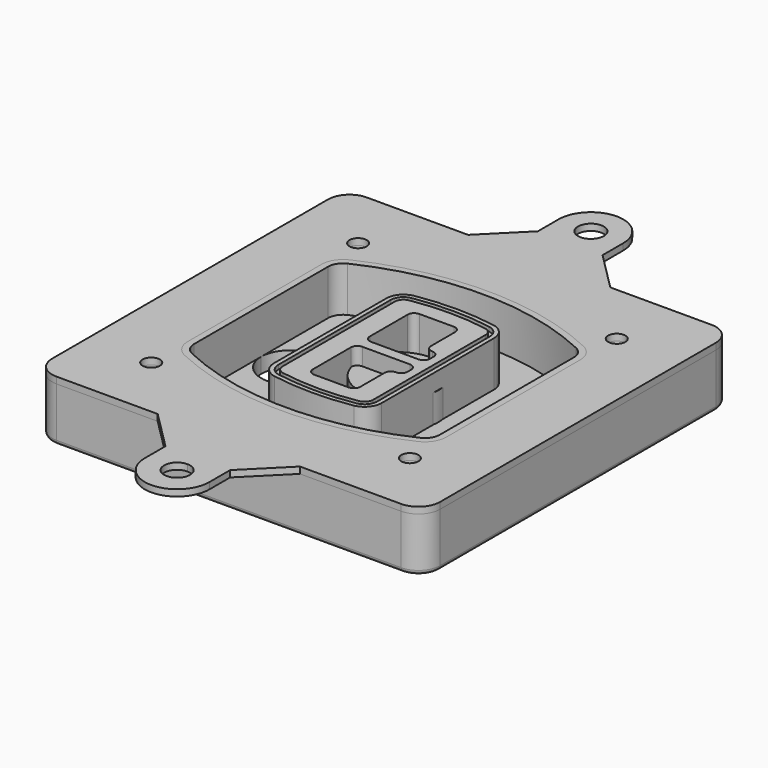
from build123d import *

# Parameters (mm, degrees)
F0_R      = 4
F1_DEPTH  = 25
F2_DEPTH  = 3
F3_DEPTH  = 18
F5_DEPTH  = 21
F6_DEPTH  = 2
F8_DEPTH  = 20
F9_DEPTH  = 16
F10_DEPTH = 25
F7_R      = 6
F7_R_2    = 4
F11_DEPTH = 6
F13_DEPTH = 9
F15_R     = 2
F16_R     = 6
F16_R_2   = 4
F17_DEPTH = 3


# Not quite as in the source:
# - a feature of the source that left no trace in its solid (it failed there, or was rolled back) is left out
# - a feature names something its author has since deleted; it is built from what else it names


with BuildPart() as f1:
    # F0 (on Top) → F1 (new body)
    with BuildSketch(Plane.XY):
        with BuildLine():
            ThreePointArc((-90, -80), (-87.0710678119, -87.0710678119), (-80, -90))
            Line((-80, -90), (80, -90))
            ThreePointArc((80, -90), (87.0710678119, -87.0710678119), (90, -80))
            Line((90, -80), (90, 80))
            ThreePointArc((90, 80), (87.0710678119, 87.0710678119), (80, 90))
            Line((80, 90), (-80, 90))
            ThreePointArc((-80, 90), (-87.0710678119, 87.0710678119), (-90, 80))
            Line((-90, 80), (-90, -80))
        make_face()
        with Locations((-60, -60)):
            Circle(F0_R, mode=Mode.SUBTRACT)
        with Locations((60, -60)):
            Circle(F0_R, mode=Mode.SUBTRACT)
        with Locations((-60, 60)):
            Circle(F0_R, mode=Mode.SUBTRACT)
        with BuildLine():
            ThreePointArc((-64, 38.8308515907), (-61.8195654598, 46.3340424013), (-55.9574468085, 51.5000594398))
            ThreePointArc((-55.9574468085, 51.5000594398), (0, 64), (55.9574468085, 51.5000594398))
            ThreePointArc((55.9574468085, 51.5000594398), (61.8195654598, 46.3340424013), (64, 38.8308515907))
            Line((64, 38.8308515907), (64, -38.8308515907))
            ThreePointArc((64, -38.8308515907), (61.8195654598, -46.3340424013), (55.9574468085, -51.5000594398))
            ThreePointArc((55.9574468085, -51.5000594398), (0, -64), (-55.9574468085, -51.5000594398))
            ThreePointArc((-55.9574468085, -51.5000594398), (-61.8195654598, -46.3340424013), (-64, -38.8308515907))
            Line((-64, -38.8308515907), (-64, 38.8308515907))
        make_face(mode=Mode.SUBTRACT)
        with Locations((60, 60)):
            Circle(F0_R, mode=Mode.SUBTRACT)
        with BuildLine():
            ThreePointArc((55.9574468085, 51.5000594398), (0, 64), (-55.9574468085, 51.5000594398))
            ThreePointArc((-55.9574468085, 51.5000594398), (-61.8195654598, 46.3340424013), (-64, 38.8308515907))
            Line((-64, 38.8308515907), (-64, -38.8308515907))
            ThreePointArc((-64, -38.8308515907), (-61.8195654598, -46.3340424013), (-55.9574468085, -51.5000594398))
            ThreePointArc((-55.9574468085, -51.5000594398), (0, -64), (55.9574468085, -51.5000594398))
            ThreePointArc((55.9574468085, -51.5000594398), (61.8195654598, -46.3340424013), (64, -38.8308515907))
            Line((64, -38.8308515907), (64, 38.8308515907))
            ThreePointArc((64, 38.8308515907), (61.8195654598, 46.3340424013), (55.9574468085, 51.5000594398))
        make_face()
        with BuildLine():
            Line((-60, -38.8308515907), (-60, 38.8308515907))
            ThreePointArc((-60, 38.8308515907), (-58.442546757, 44.1902735983), (-54.2553191489, 47.8802857686))
            ThreePointArc((-54.2553191489, 47.8802857686), (0, 60), (54.2553191489, 47.8802857686))
            ThreePointArc((54.2553191489, 47.8802857686), (58.442546757, 44.1902735983), (60, 38.8308515907))
            Line((60, 38.8308515907), (60, -38.8308515907))
            ThreePointArc((60, -38.8308515907), (58.442546757, -44.1902735983), (54.2553191489, -47.8802857686))
            ThreePointArc((54.2553191489, -47.8802857686), (0, -60), (-54.2553191489, -47.8802857686))
            ThreePointArc((-54.2553191489, -47.8802857686), (-58.442546757, -44.1902735983), (-60, -38.8308515907))
        make_face(mode=Mode.SUBTRACT)
        with BuildLine():
            ThreePointArc((-54.2553191489, 47.8802857686), (-58.442546757, 44.1902735983), (-60, 38.8308515907))
            Line((-60, 38.8308515907), (-60, -38.8308515907))
            ThreePointArc((-60, -38.8308515907), (-58.442546757, -44.1902735983), (-54.2553191489, -47.8802857686))
            ThreePointArc((-54.2553191489, -47.8802857686), (0, -60), (54.2553191489, -47.8802857686))
            ThreePointArc((54.2553191489, -47.8802857686), (58.442546757, -44.1902735983), (60, -38.8308515907))
            Line((60, -38.8308515907), (60, 38.8308515907))
            ThreePointArc((60, 38.8308515907), (58.442546757, 44.1902735983), (54.2553191489, 47.8802857686))
            ThreePointArc((54.2553191489, 47.8802857686), (0, 60), (-54.2553191489, 47.8802857686))
        make_face()
        with BuildLine():
            ThreePointArc((52.9787234043, 45.1654555152), (55.9097827299, 42.582446996), (57, 38.8308515907))
            Line((57, 38.8308515907), (57, -38.8308515907))
            ThreePointArc((57, -38.8308515907), (55.9097827299, -42.582446996), (52.9787234043, -45.1654555152))
            ThreePointArc((52.9787234043, -45.1654555152), (0, -57), (-52.9787234043, -45.1654555152))
            ThreePointArc((-52.9787234043, -45.1654555152), (-55.9097827299, -42.582446996), (-57, -38.8308515907))
            Line((-57, -38.8308515907), (-57, 38.8308515907))
            ThreePointArc((-57, 38.8308515907), (-55.9097827299, 42.582446996), (-52.9787234043, 45.1654555152))
            ThreePointArc((-52.9787234043, 45.1654555152), (0, 57), (52.9787234043, 45.1654555152))
        make_face(mode=Mode.SUBTRACT)
        with BuildLine():
            Line((57, -38.8308515907), (57, 38.8308515907))
            ThreePointArc((57, 38.8308515907), (55.9097827299, 42.582446996), (52.9787234043, 45.1654555152))
            ThreePointArc((52.9787234043, 45.1654555152), (0, 57), (-52.9787234043, 45.1654555152))
            ThreePointArc((-52.9787234043, 45.1654555152), (-55.9097827299, 42.582446996), (-57, 38.8308515907))
            Line((-57, 38.8308515907), (-57, -38.8308515907))
            ThreePointArc((-57, -38.8308515907), (-55.9097827299, -42.582446996), (-52.9787234043, -45.1654555152))
            ThreePointArc((-52.9787234043, -45.1654555152), (0, -57), (52.9787234043, -45.1654555152))
            ThreePointArc((52.9787234043, -45.1654555152), (55.9097827299, -42.582446996), (57, -38.8308515907))
        make_face()
    extrude(amount=-F1_DEPTH)

    # F0 (on Top) → F2 (join)
    with BuildSketch(Plane.XY):
        with BuildLine():
            ThreePointArc((-54.2553191489, 47.8802857686), (-58.442546757, 44.1902735983), (-60, 38.8308515907))
            Line((-60, 38.8308515907), (-60, -38.8308515907))
            ThreePointArc((-60, -38.8308515907), (-58.442546757, -44.1902735983), (-54.2553191489, -47.8802857686))
            ThreePointArc((-54.2553191489, -47.8802857686), (0, -60), (54.2553191489, -47.8802857686))
            ThreePointArc((54.2553191489, -47.8802857686), (58.442546757, -44.1902735983), (60, -38.8308515907))
            Line((60, -38.8308515907), (60, 38.8308515907))
            ThreePointArc((60, 38.8308515907), (58.442546757, 44.1902735983), (54.2553191489, 47.8802857686))
            ThreePointArc((54.2553191489, 47.8802857686), (0, 60), (-54.2553191489, 47.8802857686))
        make_face()
        with BuildLine():
            ThreePointArc((52.9787234043, 45.1654555152), (55.9097827299, 42.582446996), (57, 38.8308515907))
            Line((57, 38.8308515907), (57, -38.8308515907))
            ThreePointArc((57, -38.8308515907), (55.9097827299, -42.582446996), (52.9787234043, -45.1654555152))
            ThreePointArc((52.9787234043, -45.1654555152), (0, -57), (-52.9787234043, -45.1654555152))
            ThreePointArc((-52.9787234043, -45.1654555152), (-55.9097827299, -42.582446996), (-57, -38.8308515907))
            Line((-57, -38.8308515907), (-57, 38.8308515907))
            ThreePointArc((-57, 38.8308515907), (-55.9097827299, 42.582446996), (-52.9787234043, 45.1654555152))
            ThreePointArc((-52.9787234043, 45.1654555152), (0, 57), (52.9787234043, 45.1654555152))
        make_face(mode=Mode.SUBTRACT)
    extrude(amount=F2_DEPTH)

    # F0 (on Top) → F3 (cut)
    with BuildSketch(Plane.XY):
        with BuildLine():
            Line((57, -38.8308515907), (57, 38.8308515907))
            ThreePointArc((57, 38.8308515907), (55.9097827299, 42.582446996), (52.9787234043, 45.1654555152))
            ThreePointArc((52.9787234043, 45.1654555152), (0, 57), (-52.9787234043, 45.1654555152))
            ThreePointArc((-52.9787234043, 45.1654555152), (-55.9097827299, 42.582446996), (-57, 38.8308515907))
            Line((-57, 38.8308515907), (-57, -38.8308515907))
            ThreePointArc((-57, -38.8308515907), (-55.9097827299, -42.582446996), (-52.9787234043, -45.1654555152))
            ThreePointArc((-52.9787234043, -45.1654555152), (0, -57), (52.9787234043, -45.1654555152))
            ThreePointArc((52.9787234043, -45.1654555152), (55.9097827299, -42.582446996), (57, -38.8308515907))
        make_face()
    extrude(amount=-F3_DEPTH, mode=Mode.SUBTRACT)

    # F4 (on face) → F5 (join, through all)
    with BuildSketch(Plane.XY.offset(3)):
        with BuildLine():
            ThreePointArc((-25, -32.5662280692), (-23.1122504785, -37.7276614059), (-18.3399014778, -40.4532214146))
            ThreePointArc((-18.3399014778, -40.4532214146), (0, -42), (18.3399014778, -40.4532214146))
            ThreePointArc((18.3399014778, -40.4532214146), (23.1122504785, -37.7276614059), (25, -32.5662280692))
            Line((25, -32.5662280692), (25, 32.5662280692))
            ThreePointArc((25, 32.5662280692), (23.1122504785, 37.7276614059), (18.3399014778, 40.4532214146))
            ThreePointArc((18.3399014778, 40.4532214146), (0, 42), (-18.3399014778, 40.4532214146))
            ThreePointArc((-18.3399014778, 40.4532214146), (-23.1122504785, 37.7276614059), (-25, 32.5662280692))
            Line((-25, 32.5662280692), (-25, -32.5662280692))
        make_face()
        with BuildLine():
            ThreePointArc((18.0049261084, 38.4814730782), (21.5841878588, 36.4373030717), (23, 32.5662280692))
            Line((23, 32.5662280692), (23, -32.5662280692))
            ThreePointArc((23, -32.5662280692), (21.5841878588, -36.4373030717), (18.0049261084, -38.4814730782))
            ThreePointArc((18.0049261084, -38.4814730782), (0, -40), (-18.0049261084, -38.4814730782))
            ThreePointArc((-18.0049261084, -38.4814730782), (-21.5841878588, -36.4373030717), (-23, -32.5662280692))
            Line((-23, -32.5662280692), (-23, 32.5662280692))
            ThreePointArc((-23, 32.5662280692), (-21.5841878588, 36.4373030717), (-18.0049261084, 38.4814730782))
            ThreePointArc((-18.0049261084, 38.4814730782), (0, 40), (18.0049261084, 38.4814730782))
        make_face(mode=Mode.SUBTRACT)
        with BuildLine():
            Line((23, -32.5662280692), (23, 32.5662280692))
            ThreePointArc((23, 32.5662280692), (21.5841878588, 36.4373030717), (18.0049261084, 38.4814730782))
            ThreePointArc((18.0049261084, 38.4814730782), (0, 40), (-18.0049261084, 38.4814730782))
            ThreePointArc((-18.0049261084, 38.4814730782), (-21.5841878588, 36.4373030717), (-23, 32.5662280692))
            Line((-23, 32.5662280692), (-23, -32.5662280692))
            ThreePointArc((-23, -32.5662280692), (-21.5841878588, -36.4373030717), (-18.0049261084, -38.4814730782))
            ThreePointArc((-18.0049261084, -38.4814730782), (0, -40), (18.0049261084, -38.4814730782))
            ThreePointArc((18.0049261084, -38.4814730782), (21.5841878588, -36.4373030717), (23, -32.5662280692))
        make_face()
        with BuildLine():
            ThreePointArc((17.6699507389, 36.5097247419), (20.0561252392, 35.1469447375), (21, 32.5662280692))
            Line((21, 32.5662280692), (21, -32.5662280692))
            ThreePointArc((21, -32.5662280692), (20.0561252392, -35.1469447375), (17.6699507389, -36.5097247419))
            ThreePointArc((17.6699507389, -36.5097247419), (0, -38), (-17.6699507389, -36.5097247419))
            ThreePointArc((-17.6699507389, -36.5097247419), (-20.0561252392, -35.1469447375), (-21, -32.5662280692))
            Line((-21, -32.5662280692), (-21, 32.5662280692))
            ThreePointArc((-21, 32.5662280692), (-20.0561252392, 35.1469447375), (-17.6699507389, 36.5097247419))
            ThreePointArc((-17.6699507389, 36.5097247419), (0, 38), (17.6699507389, 36.5097247419))
        make_face(mode=Mode.SUBTRACT)
        with BuildLine():
            Line((21, -32.5662280692), (21, 32.5662280692))
            ThreePointArc((21, 32.5662280692), (20.0561252392, 35.1469447375), (17.6699507389, 36.5097247419))
            ThreePointArc((17.6699507389, 36.5097247419), (0, 38), (-17.6699507389, 36.5097247419))
            ThreePointArc((-17.6699507389, 36.5097247419), (-20.0561252392, 35.1469447375), (-21, 32.5662280692))
            Line((-21, 32.5662280692), (-21, -32.5662280692))
            ThreePointArc((-21, -32.5662280692), (-20.0561252392, -35.1469447375), (-17.6699507389, -36.5097247419))
            ThreePointArc((-17.6699507389, -36.5097247419), (0, -38), (17.6699507389, -36.5097247419))
            ThreePointArc((17.6699507389, -36.5097247419), (20.0561252392, -35.1469447375), (21, -32.5662280692))
        make_face()
        with BuildLine():
            Line((-8, -2.5), (14, -2.5))
            ThreePointArc((14, -2.5), (16.1213203436, -3.3786796564), (17, -5.5))
            Line((17, -5.5), (17, -7.5))
            ThreePointArc((17, -7.5), (16.1213203436, -9.6213203436), (14, -10.5))
            ThreePointArc((14, -10.5), (11.8786796564, -11.3786796564), (11, -13.5))
            Line((11, -13.5), (11, -27.5))
            ThreePointArc((11, -27.5), (10.1213203436, -29.6213203436), (8, -30.5))
            Line((8, -30.5), (-8, -30.5))
            ThreePointArc((-8, -30.5), (-10.1213203436, -29.6213203436), (-11, -27.5))
            Line((-11, -27.5), (-11, -5.5))
            ThreePointArc((-11, -5.5), (-10.1213203436, -3.3786796564), (-8, -2.5))
        make_face(mode=Mode.SUBTRACT)
        with BuildLine():
            ThreePointArc((-8, 2.5), (-10.1213203436, 3.3786796564), (-11, 5.5))
            Line((-11, 5.5), (-11, 27.5))
            ThreePointArc((-11, 27.5), (-10.1213203436, 29.6213203436), (-8, 30.5))
            Line((-8, 30.5), (8, 30.5))
            ThreePointArc((8, 30.5), (10.1213203436, 29.6213203436), (11, 27.5))
            Line((11, 27.5), (11, 13.5))
            ThreePointArc((11, 13.5), (11.8786796564, 11.3786796564), (14, 10.5))
            ThreePointArc((14, 10.5), (16.1213203436, 9.6213203436), (17, 7.5))
            Line((17, 7.5), (17, 5.5))
            ThreePointArc((17, 5.5), (16.1213203436, 3.3786796564), (14, 2.5))
            Line((14, 2.5), (-8, 2.5))
        make_face(mode=Mode.SUBTRACT)
    extrude(amount=-F5_DEPTH)

    # F4 (on face) → F6 (cut)
    with BuildSketch(Plane.XY.offset(3)):
        with BuildLine():
            Line((23, -32.5662280692), (23, 32.5662280692))
            ThreePointArc((23, 32.5662280692), (21.5841878588, 36.4373030717), (18.0049261084, 38.4814730782))
            ThreePointArc((18.0049261084, 38.4814730782), (0, 40), (-18.0049261084, 38.4814730782))
            ThreePointArc((-18.0049261084, 38.4814730782), (-21.5841878588, 36.4373030717), (-23, 32.5662280692))
            Line((-23, 32.5662280692), (-23, -32.5662280692))
            ThreePointArc((-23, -32.5662280692), (-21.5841878588, -36.4373030717), (-18.0049261084, -38.4814730782))
            ThreePointArc((-18.0049261084, -38.4814730782), (0, -40), (18.0049261084, -38.4814730782))
            ThreePointArc((18.0049261084, -38.4814730782), (21.5841878588, -36.4373030717), (23, -32.5662280692))
        make_face()
        with BuildLine():
            ThreePointArc((17.6699507389, 36.5097247419), (20.0561252392, 35.1469447375), (21, 32.5662280692))
            Line((21, 32.5662280692), (21, -32.5662280692))
            ThreePointArc((21, -32.5662280692), (20.0561252392, -35.1469447375), (17.6699507389, -36.5097247419))
            ThreePointArc((17.6699507389, -36.5097247419), (0, -38), (-17.6699507389, -36.5097247419))
            ThreePointArc((-17.6699507389, -36.5097247419), (-20.0561252392, -35.1469447375), (-21, -32.5662280692))
            Line((-21, -32.5662280692), (-21, 32.5662280692))
            ThreePointArc((-21, 32.5662280692), (-20.0561252392, 35.1469447375), (-17.6699507389, 36.5097247419))
            ThreePointArc((-17.6699507389, 36.5097247419), (0, 38), (17.6699507389, 36.5097247419))
        make_face(mode=Mode.SUBTRACT)
    extrude(amount=-F6_DEPTH, mode=Mode.SUBTRACT)

    # F7 (on face) → F8 (join)
    with BuildSketch(Plane(origin=(0, 0, -25), x_dir=(1, 0, 0), z_dir=(0, 0, -1))):
        with BuildLine():
            ThreePointArc((-6.71157564, 0), (6.7567035675, 13.4682792075), (20.224982775, 0))
            Line((20.224982775, 0), (25.224982775, 0))
            ThreePointArc((25.224982775, 0), (6.7567035675, 18.4682792075), (-11.71157564, 0))
            Line((-11.71157564, 0), (-6.71157564, 0))
        make_face()
        with BuildLine():
            Line((-6.71157564, 0), (20.224982775, 0))
            ThreePointArc((20.224982775, 0), (6.7567035675, 13.4682792075), (-6.71157564, 0))
        make_face()
        with BuildLine():
            ThreePointArc((-6.71157564, 0), (6.7567035675, -13.4682792075), (20.224982775, 0))
            Line((20.224982775, 0), (-6.71157564, 0))
        make_face()
        with BuildLine():
            Line((25.224982775, 0), (20.224982775, 0))
            ThreePointArc((20.224982775, 0), (6.7567035675, -13.4682792075), (-6.71157564, 0))
            Line((-6.71157564, 0), (-11.71157564, 0))
            ThreePointArc((-11.71157564, 0), (6.7567035675, -18.4682792075), (25.224982775, 0))
        make_face()
    extrude(amount=-F8_DEPTH)

    # F7 (on face) → F9 (cut)
    with BuildSketch(Plane(origin=(0, 0, -25), x_dir=(1, 0, 0), z_dir=(0, 0, -1))):
        with BuildLine():
            Line((-6.71157564, 0), (20.224982775, 0))
            ThreePointArc((20.224982775, 0), (6.7567035675, 13.4682792075), (-6.71157564, 0))
        make_face()
        with BuildLine():
            ThreePointArc((-6.71157564, 0), (6.7567035675, -13.4682792075), (20.224982775, 0))
            Line((20.224982775, 0), (-6.71157564, 0))
        make_face()
    extrude(amount=-F9_DEPTH, mode=Mode.SUBTRACT)

    # F7 (on face) → F10 (cut)
    with BuildSketch(Plane(origin=(0, 0, -25), x_dir=(1, 0, 0), z_dir=(0, 0, -1))):
        with BuildLine():
            Line((-57, 0), (-30.0634415849, 0))
            ThreePointArc((-30.0634415849, 0), (-43.5317207925, 13.4682792075), (-57, 0))
        make_face()
        with BuildLine():
            ThreePointArc((-57, 0), (-43.5317207925, -13.4682792075), (-30.0634415849, 0))
            Line((-30.0634415849, 0), (-57, 0))
        make_face()
    extrude(amount=-F10_DEPTH, mode=Mode.SUBTRACT)

    # F7 (on face) → F11 (cut)
    with BuildSketch(Plane(origin=(0, 0, -25), x_dir=(1, 0, 0), z_dir=(0, 0, -1))):
        with Locations((60, -60)):
            Circle(F7_R)
        with Locations((60, -60)):
            Circle(F7_R_2, mode=Mode.SUBTRACT)
        with Locations((-60, -60)):
            Circle(F7_R)
        with Locations((-60, -60)):
            Circle(F7_R_2, mode=Mode.SUBTRACT)
        with Locations((-60, 60)):
            Circle(F7_R)
        with Locations((-60, 60)):
            Circle(F7_R_2, mode=Mode.SUBTRACT)
        with Locations((60, 60)):
            Circle(F7_R)
        with Locations((60, 60)):
            Circle(F7_R_2, mode=Mode.SUBTRACT)
    extrude(amount=-F11_DEPTH, mode=Mode.SUBTRACT)

    # F12 (on face) → F13 (cut, through all)
    with BuildSketch(Plane(origin=(0, 0, -9), x_dir=(1, 0, 0), z_dir=(0, 0, -1))):
        with BuildLine():
            ThreePointArc((20.224982775, 0), (20.1663399806, 1.2554664788), (19.9909222755, 2.5))
            Line((19.9909222755, 2.5), (14, 2.5))
            ThreePointArc((14, 2.5), (16.1213203436, 3.3786796564), (17, 5.5))
            Line((17, 5.5), (17, 7.5))
            ThreePointArc((17, 7.5), (16.1213203436, 9.6213203436), (14, 10.5))
            ThreePointArc((14, 10.5), (12.1627255951, 11.1284134507), (11.0951631559, 12.750384826))
            ThreePointArc((11.0951631559, 12.750384826), (11.0476113807, 12.7664660322), (11, 12.7823698976))
            Line((11, 12.7823698976), (11, -12.7823698976))
            ThreePointArc((11, -12.7823698976), (11.0476113807, -12.7664660322), (11.0951631559, -12.750384826))
            ThreePointArc((11.0951631559, -12.750384826), (12.1627255951, -11.1284134507), (14, -10.5))
            ThreePointArc((14, -10.5), (16.1213203436, -9.6213203436), (17, -7.5))
            Line((17, -7.5), (17, -5.5))
            ThreePointArc((17, -5.5), (16.1213203436, -3.3786796564), (14, -2.5))
            Line((14, -2.5), (19.9909222755, -2.5))
            ThreePointArc((19.9909222755, -2.5), (20.1663399806, -1.2554664788), (20.224982775, 0))
        make_face()
    extrude(amount=F13_DEPTH, mode=Mode.SUBTRACT)

    # F15
    f15_edges = [f1.edges().sort_by_distance(p)[0] for p in [
        (0, -90, -25),
        (-87.071068, -87.071068, -25),
        (-90, 0, -25),
        (-87.071068, 87.071068, -25),
        (87.071068, -87.071068, -25),
        (0, 90, -25),
        (90, 0, -25),
        (87.071068, 87.071068, -25),
    ]]
    fillet(f15_edges, radius=F15_R)


with BuildPart() as f17:
    # F16 (on face) → F17 (new body, through all)
    with BuildSketch(Plane.XY):
        with BuildLine():
            Line((-15, 108), (-33, 90))
            Line((-33, 90), (33, 90))
            Line((33, 90), (15, 108))
            Line((15, 108), (15, 120))
            ThreePointArc((15, 120), (0, 135), (-15, 120))
            Line((-15, 120), (-15, 108))
        make_face()
        with Locations((0, 120)):
            Circle(F16_R, mode=Mode.SUBTRACT)
        with BuildLine():
            Line((0, -90), (-33, -90))
            Line((-33, -90), (-15, -108))
            Line((-15, -108), (-15, -120))
            ThreePointArc((-15, -120), (0, -135), (15, -120))
            Line((15, -120), (15, -108))
            Line((15, -108), (33, -90))
            Line((33, -90), (0, -90))
        make_face()
        with BuildLine():
            ThreePointArc((6, -120), (-4.2426406871, -124.2426406871), (0, -114))
            ThreePointArc((0, -114), (4.2426406871, -115.7573593129), (6, -120))
        make_face(mode=Mode.SUBTRACT)
        with BuildLine():
            Line((33, 90), (-33, 90))
            Line((-33, 90), (-80, 90))
            ThreePointArc((-80, 90), (-87.0710678119, 87.0710678119), (-90, 80))
            Line((-90, 80), (-90, -80))
            ThreePointArc((-90, -80), (-87.0710678119, -87.0710678119), (-80, -90))
            Line((-80, -90), (-33, -90))
            Line((-33, -90), (0, -90))
            Line((0, -90), (33, -90))
            Line((33, -90), (80, -90))
            ThreePointArc((80, -90), (87.0710678119, -87.0710678119), (90, -80))
            Line((90, -80), (90, 80))
            ThreePointArc((90, 80), (87.0710678119, 87.0710678119), (80, 90))
            Line((80, 90), (33, 90))
        make_face()
        with Locations((-60, -60)):
            Circle(F16_R_2, mode=Mode.SUBTRACT)
        with Locations((60, -60)):
            Circle(F16_R_2, mode=Mode.SUBTRACT)
        with Locations((-60, 60)):
            Circle(F16_R_2, mode=Mode.SUBTRACT)
        with BuildLine():
            ThreePointArc((-60, 38.8308515907), (-58.442546757, 44.1902735983), (-54.2553191489, 47.8802857686))
            ThreePointArc((-54.2553191489, 47.8802857686), (0, 60), (54.2553191489, 47.8802857686))
            ThreePointArc((54.2553191489, 47.8802857686), (58.442546757, 44.1902735983), (60, 38.8308515907))
            Line((60, 38.8308515907), (60, -38.8308515907))
            ThreePointArc((60, -38.8308515907), (58.442546757, -44.1902735983), (54.2553191489, -47.8802857686))
            ThreePointArc((54.2553191489, -47.8802857686), (0, -60), (-54.2553191489, -47.8802857686))
            ThreePointArc((-54.2553191489, -47.8802857686), (-58.442546757, -44.1902735983), (-60, -38.8308515907))
            Line((-60, -38.8308515907), (-60, 38.8308515907))
        make_face(mode=Mode.SUBTRACT)
        with Locations((60, 60)):
            Circle(F16_R_2, mode=Mode.SUBTRACT)
    extrude(amount=F17_DEPTH)


solid = Compound([f1.part, f17.part])
